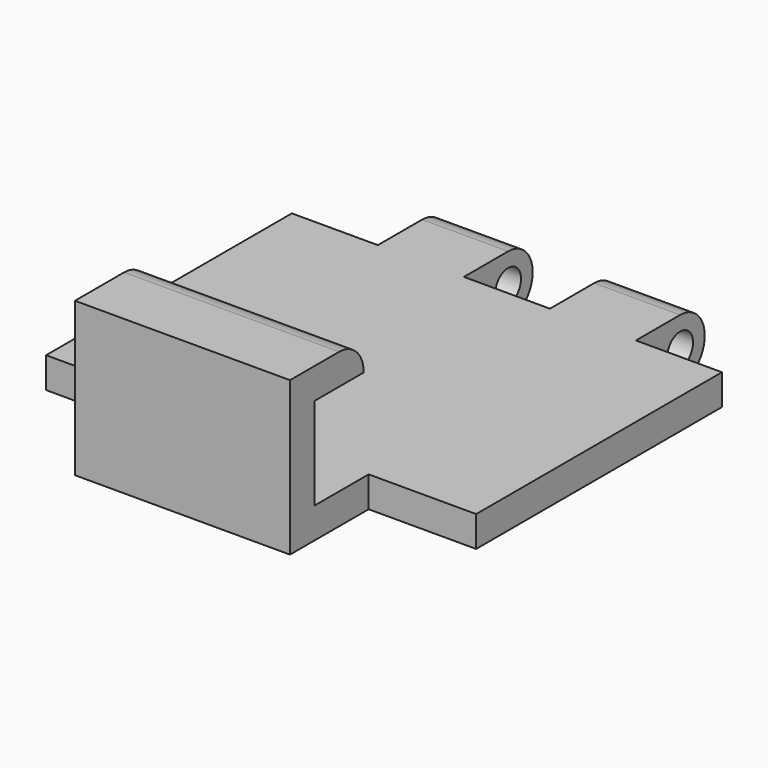
from build123d import *

# Parameters (mm, degrees)
F0_R          = 2.625
F1_DEPTH      = 70
F2_W          = 17.5
F2_H          = 25
F3_DEPTH      = 16
F5_W          = 14
F5_H          = 10
F6_DEPTH      = 9
F6_DEPTH_BACK = 5.001
F7_R          = 4.99999
F8_ANGLE      = 180
F9_ANGLE      = 180


# Not quite as in the source:
# - a fillet or chamfer is up to 0.001 mm smaller than in the source, because OpenCascade refuses the exact size


with BuildPart() as f1:
    # F0 (on Right) → F1 (new body)
    with BuildSketch(Plane.YZ):
        with BuildLine():
            Line((-5, 5), (-20.3439258039, 5))
            Line((-20.3439258039, 5), (-75, 5))
            ThreePointArc((-75, 5), (-79.3301270189, -2.5), (-70.6698729811, -2.5))
            ThreePointArc((-70.6698729811, -2.5), (-68.8397459622, -0.6698729811), (-66.3397459622, 0))
            Line((-66.3397459622, 0), (0, 0))
            Line((0, 0), (0, 5))
            Line((0, 5), (0, 25))
            Line((0, 25), (-15, 25))
            Line((-15, 25), (-15, 20))
            Line((-15, 20), (-5, 20))
            Line((-5, 20), (-5, 5))
        make_face()
        with Locations((-75, 0)):
            Circle(F0_R, mode=Mode.SUBTRACT)
    extrude(amount=F1_DEPTH)

    # F2 (on Front) → F3 (cut)
    with BuildSketch(Plane.XZ):
        with Locations((8.75, 12.5)):
            Rectangle(F2_W, F2_H)
        with Locations((61.25, 12.5)):
            Rectangle(F2_W, F2_H)
    extrude(amount=F3_DEPTH, mode=Mode.SUBTRACT)

    # F5 (on offset) → F6 (cut, two sides)
    with BuildSketch(Plane.XZ.offset(75)) as f6_sk:
        with Locations((7, 0)):
            Rectangle(F5_W, F5_H)
        with Locations((35, 0)):
            Rectangle(F5_W, F5_H)
        with Locations((63, 0)):
            Rectangle(F5_W, F5_H)
    extrude(amount=-F6_DEPTH, mode=Mode.SUBTRACT)
    extrude(f6_sk.sketch, amount=F6_DEPTH_BACK, mode=Mode.SUBTRACT)

    # F7 (radius 5 in the source; OpenCascade refuses exactly that, so slightly less here)
    f7_edges = [f1.edges().sort_by_distance(p)[0] for p in [
        (35, -15, 25),
    ]]
    fillet(f7_edges, radius=F7_R)


with BuildPart() as f1_1:
    # F8: moved
    add(f1.part.rotate(Axis((56, -75, 0), (-1, 0, 0)), F8_ANGLE))


with BuildPart() as f1_2:
    # F9: moved
    add(f1_1.part.rotate(Axis((70, -109, 0), (0, -1, 0)), F9_ANGLE))


solid = f1_2.part
